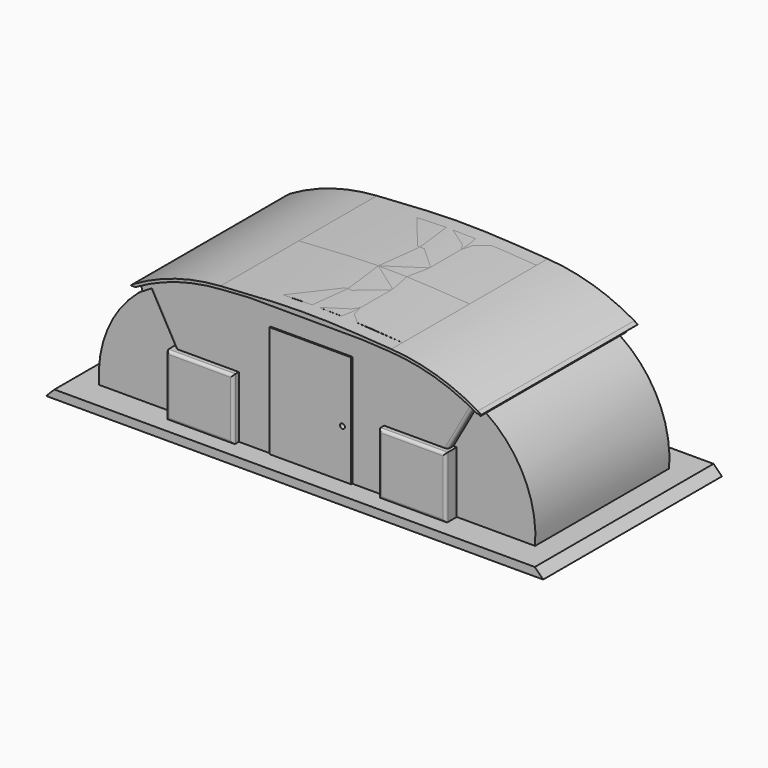
from build123d import *

# Parameters (mm, degrees)
F0_W        = 73.01958814
F0_H        = 200
F0_R        = 4.4064886868
F1_DEPTH    = 150
F2_DEPTH    = 175
F3_DEPTH    = 175
F4_DEPTH    = 162.5
F5_DEPTH    = 165
F6_R        = 5
F6_2_R      = 5
F6_3_R      = 5
F7_W        = 900
F7_H        = 400
F7_W_2      = 780.6288967379
F7_H_2      = 300
F8_DEPTH    = 15
F9_T1_DEPTH = 502.8673195186
F10_DEPTH   = 15


# Not quite as in the source:
# - a fillet or chamfer that OpenCascade refuses, or shapes differently, is made with other operations: its cross-section is extruded or revolved along the edge and cut away or added
# - ends of sketch curves that miss each other by under 0.0002 mm in the source are joined


with BuildPart() as f1:
    # F0 (on Front) → F1 (new body, symmetric)
    with BuildSketch(Plane.XZ):
        with BuildLine():
            Line((73.2485631082, 199.8381957412), (73.2485631082, -0.1618042588))
            Line((73.2485631082, -0.1618042588), (130.2289748106, -0.1618042588))
            Line((130.2289748106, -0.1618042588), (130.2289749682, 109.8381957412))
            Line((130.2289749682, 109.8381957412), (244.361110868, 109.8381957412))
            Line((244.361110868, 109.8381957412), (288.9051257209, 189.2969646801))
            ThreePointArc((288.9051257209, 189.2969646801), (295.915659625, 185.1774143178), (302.7529489944, 180.7763059474))
            Line((302.7529489944, 180.7763059474), (305.6783307484, 191.6270836714))
            ThreePointArc((305.6783307484, 191.6270836714), (230.6863223559, 224.0165542057), (150.2289749682, 238.1408019938))
            Line((150.2289749682, 238.1408019938), (102.1122379409, 240.8775282261))
            Line((102.1122379409, 240.8775282261), (-101.8451842253, 241.4292395115))
            Line((-101.8451842253, 241.4292395115), (-151.505661922, 238.0378207475))
            ThreePointArc((-151.505661922, 238.0378207475), (-231.0604446139, 223.7664550341), (-305.220380812, 191.6270836714))
            Line((-305.220380812, 191.6270836714), (-302.294999058, 180.7763059474))
            ThreePointArc((-302.294999058, 180.7763059474), (-295.4577096886, 185.1774143178), (-288.4471757845, 189.2969646801))
            Line((-288.4471757845, 189.2969646801), (-243.9031609316, 109.8381957412))
            Line((-243.9031609316, 109.8381957412), (-129.7710250318, 109.8381957412))
            Line((-129.7710250318, 109.8381957412), (-129.7710250318, -0.1618042588))
            Line((-129.7710250318, -0.1618042588), (-72.7906131718, -0.1618042588))
            Line((-72.7906131718, -0.1618042588), (-72.7906131718, 199.8381957412))
            Line((-72.7906131718, 199.8381957412), (0.2289749682, 199.8381957412))
            Line((0.2289749682, 199.8381957412), (73.2485631082, 199.8381957412))
        make_face()
        Polygon((-249.7710250318, -0.1618042588), (-129.7710250318, -0.1618042588), (-129.7710250318, 109.8381957412), (-243.9031609316, 109.8381957412), (-249.7710250318, 109.8381957412), (-249.7710250318, 46.5387346062), align=None)
        with BuildLine():
            Line((-366.9111720315, 109.3456217277), (-249.7710250318, 46.5387346062))
            Line((-249.7710250318, 46.5387346062), (-249.7710250318, 109.8381957412))
            Line((-249.7710250318, 109.8381957412), (-243.9031609316, 109.8381957412))
            Line((-243.9031609316, 109.8381957412), (-288.4471757845, 189.2969646801))
            ThreePointArc((-288.4471757845, 189.2969646801), (-295.4577096886, 185.1774143178), (-302.294999058, 180.7763059474))
            ThreePointArc((-302.294999058, 180.7763059474), (-338.967392604, 149.0089145388), (-366.9111720315, 109.3456217277))
        make_face()
        with BuildLine():
            Line((-390.0854734008, -0.1618042588), (-249.7710250318, -0.1618042588))
            Line((-249.7710250318, -0.1618042588), (-249.7710250318, 46.5387346062))
            Line((-249.7710250318, 46.5387346062), (-366.9111720315, 109.3456217277))
            ThreePointArc((-366.9111720315, 109.3456217277), (-386.3153062929, 56.2461630608), (-390.0854734008, -0.1618042588))
        make_face()
        with Locations((36.7387690382, 99.8381957412)):
            Rectangle(F0_W, F0_H)
        with Locations((57.5472824275, 86.3982066512)):
            Circle(F0_R, mode=Mode.SUBTRACT)
        with Locations((-36.2808191018, 99.8381957412)):
            Rectangle(F0_W, F0_H)
        with BuildLine():
            Line((288.9051257209, 189.2969646801), (244.361110868, 109.8381957412))
            Line((244.361110868, 109.8381957412), (250.2289749682, 109.8381957412))
            Line((250.2289749682, 109.8381957412), (250.2289749682, 46.5387346062))
            Line((250.2289749682, 46.5387346062), (367.3691219679, 109.3456217277))
            ThreePointArc((367.3691219679, 109.3456217277), (339.4253425404, 149.0089145388), (302.7529489944, 180.7763059474))
            ThreePointArc((302.7529489944, 180.7763059474), (295.915659625, 185.1774143178), (288.9051257209, 189.2969646801))
        make_face()
        with BuildLine():
            Line((250.2289749682, 46.5387346062), (250.2289749682, -0.1618042588))
            Line((250.2289749682, -0.1618042588), (390.5434233372, -0.1618042588))
            ThreePointArc((390.5434233372, -0.1618042588), (386.7732562293, 56.2461630608), (367.3691219679, 109.3456217277))
            Line((367.3691219679, 109.3456217277), (250.2289749682, 46.5387346062))
        make_face()
        with BuildLine():
            Line((130.2289749682, 109.8381957412), (130.2289749682, -0.1618042588))
            Line((130.2289749682, -0.1618042588), (190.2289749682, -0.1618042588))
            Line((190.2289749682, -0.1618042588), (191.104793533, -0.1618042588))
            Line((191.104793533, -0.1618042588), (191.104793533, 2.3381956821))
            ThreePointArc((191.104793533, 2.3381956821), (179.0104848205, 17.996944923), (197.2172556875, 25.7417641993))
            ThreePointArc((197.2172556875, 25.7417641993), (200.0262220751, 23.5936575642), (202.1212084331, 20.7448531759))
            Line((202.1212084331, 20.7448531759), (250.2289749682, 46.5387346062))
            Line((250.2289749682, 46.5387346062), (250.2289749682, 109.8381957412))
            Line((250.2289749682, 109.8381957412), (244.361110868, 109.8381957412))
            Line((244.361110868, 109.8381957412), (130.2289749682, 109.8381957412))
        make_face()
        with BuildLine():
            ThreePointArc((197.2172556875, 25.7417641993), (179.0104848205, 17.996944923), (191.104793533, 2.3381956821))
            Line((191.104793533, 2.3381956821), (191.104793533, 14.8381956821))
            Line((191.104793533, 14.8381956821), (197.2172556875, 25.7417641993))
        make_face()
        with BuildLine():
            ThreePointArc((202.1212084331, 20.7448531759), (200.0262220751, 23.5936575642), (197.2172556875, 25.7417641993))
            Line((197.2172556875, 25.7417641993), (191.104793533, 14.8381956821))
            Line((191.104793533, 14.8381956821), (202.1212084331, 20.7448531759))
        make_face()
        with BuildLine():
            Line((191.104793533, 14.8381956821), (191.104793533, 2.3381956821))
            ThreePointArc((191.104793533, 2.3381956821), (199.9436282978, 5.9993609172), (203.604793533, 14.8381956821))
            ThreePointArc((203.604793533, 14.8381956821), (203.2282251068, 17.8832583866), (202.1212084331, 20.7448531759))
            Line((202.1212084331, 20.7448531759), (191.104793533, 14.8381956821))
        make_face()
        with BuildLine():
            Line((191.104793533, 2.3381956821), (191.104793533, -0.1618043179))
            Line((191.104793533, -0.1618042588), (250.2289749682, -0.1618042588))
            Line((250.2289749682, -0.1618042588), (250.2289749682, 46.5387346062))
            Line((250.2289749682, 46.5387346062), (202.1212084331, 20.7448531759))
            ThreePointArc((202.1212084331, 20.7448531759), (203.2282251068, 17.8832583866), (203.604793533, 14.8381956821))
            ThreePointArc((203.604793533, 14.8381956821), (199.9436282978, 5.9993609172), (191.104793533, 2.3381956821))
        make_face()
        with BuildLine():
            ThreePointArc((150.2289749682, 238.1408019938), (230.6863223559, 224.0165542057), (305.6783307484, 191.6270836714))
            Line((305.6783307484, 191.6270836714), (314.0523768961, 191.6270836714))
            Line((314.0523768961, 191.6270836714), (308.1829609782, 195.9545341232))
            ThreePointArc((308.1829609782, 195.9545341232), (233.4070394956, 228.418836004), (153.1970844362, 242.9698648181))
            add(Edge.make_bspline(
                [(-152.7391344998, 242.9698648181), (-101.8451842253, 246.5544800547), (0.018788196, 253.7290685006), (102.1122379409, 246.5580511475), (153.1970844362, 242.9698648181)],
                knots=[0, 0, 0, 0, 0.4996266007, 1, 1, 1, 1], degree=3))
            ThreePointArc((-152.7391344998, 242.9698648181), (-232.9490895592, 228.418836004), (-307.7250110418, 195.9545341232))
            Line((-307.7250110418, 195.9545341232), (-313.5944269598, 191.6270836714))
            Line((-313.5944269598, 191.6270836714), (-305.220380812, 191.6270836714))
            ThreePointArc((-305.220380812, 191.6270836714), (-231.0604446139, 223.7664550341), (-151.505661922, 238.0378207475))
            Line((-151.505661922, 238.0378207475), (-101.8451842253, 241.4292395115))
            Line((-101.8451842253, 241.4292395115), (102.1122379409, 240.8775282261))
            Line((102.1122379409, 240.8775282261), (150.2289749682, 238.1408019938))
        make_face()
    extrude(amount=F1_DEPTH, both=True)


with BuildPart() as f2:
    # F0 (on Front) → F2 (new body, symmetric)
    with BuildSketch(Plane.XZ):
        with BuildLine():
            ThreePointArc((150.2289749682, 238.1408019938), (230.6863223559, 224.0165542057), (305.6783307484, 191.6270836714))
            Line((305.6783307484, 191.6270836714), (314.0523768961, 191.6270836714))
            Line((314.0523768961, 191.6270836714), (308.1829609782, 195.9545341232))
            ThreePointArc((308.1829609782, 195.9545341232), (233.4070394956, 228.418836004), (153.1970844362, 242.9698648181))
            add(Edge.make_bspline(
                [(-152.7391344998, 242.9698648181), (-101.8451842253, 246.5544800547), (0.018788196, 253.7290685006), (102.1122379409, 246.5580511475), (153.1970844362, 242.9698648181)],
                knots=[0, 0, 0, 0, 0.4996266007, 1, 1, 1, 1], degree=3))
            ThreePointArc((-152.7391344998, 242.9698648181), (-232.9490895592, 228.418836004), (-307.7250110418, 195.9545341232))
            Line((-307.7250110418, 195.9545341232), (-313.5944269598, 191.6270836714))
            Line((-313.5944269598, 191.6270836714), (-305.220380812, 191.6270836714))
            ThreePointArc((-305.220380812, 191.6270836714), (-231.0604446139, 223.7664550341), (-151.505661922, 238.0378207475))
            Line((-151.505661922, 238.0378207475), (-101.8451842253, 241.4292395115))
            Line((-101.8451842253, 241.4292395115), (102.1122379409, 240.8775282261))
            Line((102.1122379409, 240.8775282261), (150.2289749682, 238.1408019938))
        make_face()
    extrude(amount=F2_DEPTH, both=True)


with BuildPart() as f3:
    # F0 (on Front) → F3 (new body, symmetric)
    with BuildSketch(Plane.XZ):
        Polygon((-249.7710250318, -0.1618042588), (-129.7710250318, -0.1618042588), (-129.7710250318, 109.8381957412), (-243.9031609316, 109.8381957412), (-249.7710250318, 109.8381957412), (-249.7710250318, 46.5387346062), align=None)
    extrude(amount=F3_DEPTH, both=True)

    # F6#2
    f6_2_edges = [f3.edges().sort_by_distance(p)[0] for p in [
        (-189.771025, 175, -0.161804),
        (-129.771025, 175, 54.838196),
        (-189.771025, 175, 109.838196),
        (-249.771025, 175, 54.838196),
        (-189.771025, -175, -0.161804),
        (-129.771025, -175, 54.838196),
        (-189.771025, -175, 109.838196),
        (-249.771025, -175, 54.838196),
    ]]
    fillet(f6_2_edges, radius=F6_2_R)


with BuildPart() as f3b:
    # F0 (on Front) → F3, piece 2 (new body, symmetric)
    with BuildSketch(Plane.XZ):
        with BuildLine():
            Line((130.2289749682, 109.8381957412), (130.2289749682, -0.1618042588))
            Line((130.2289749682, -0.1618042588), (190.2289749682, -0.1618042588))
            Line((190.2289749682, -0.1618042588), (191.104793533, -0.1618042588))
            Line((191.104793533, -0.1618042588), (191.104793533, 2.3381956821))
            ThreePointArc((191.104793533, 2.3381956821), (179.0104848205, 17.996944923), (197.2172556875, 25.7417641993))
            ThreePointArc((197.2172556875, 25.7417641993), (200.0262220751, 23.5936575642), (202.1212084331, 20.7448531759))
            Line((202.1212084331, 20.7448531759), (250.2289749682, 46.5387346062))
            Line((250.2289749682, 46.5387346062), (250.2289749682, 109.8381957412))
            Line((250.2289749682, 109.8381957412), (244.361110868, 109.8381957412))
            Line((244.361110868, 109.8381957412), (130.2289749682, 109.8381957412))
        make_face()
        with BuildLine():
            Line((191.104793533, 2.3381956821), (191.104793533, -0.1618043179))
            Line((191.104793533, -0.1618042588), (250.2289749682, -0.1618042588))
            Line((250.2289749682, -0.1618042588), (250.2289749682, 46.5387346062))
            Line((250.2289749682, 46.5387346062), (202.1212084331, 20.7448531759))
            ThreePointArc((202.1212084331, 20.7448531759), (203.2282251068, 17.8832583866), (203.604793533, 14.8381956821))
            ThreePointArc((203.604793533, 14.8381956821), (199.9436282978, 5.9993609172), (191.104793533, 2.3381956821))
        make_face()
        with BuildLine():
            ThreePointArc((197.2172556875, 25.7417641993), (179.0104848205, 17.996944923), (191.104793533, 2.3381956821))
            Line((191.104793533, 2.3381956821), (191.104793533, 14.8381956821))
            Line((191.104793533, 14.8381956821), (197.2172556875, 25.7417641993))
        make_face()
        with BuildLine():
            Line((191.104793533, 14.8381956821), (191.104793533, 2.3381956821))
            ThreePointArc((191.104793533, 2.3381956821), (199.9436282978, 5.9993609172), (203.604793533, 14.8381956821))
            ThreePointArc((203.604793533, 14.8381956821), (203.2282251068, 17.8832583866), (202.1212084331, 20.7448531759))
            Line((202.1212084331, 20.7448531759), (191.104793533, 14.8381956821))
        make_face()
        with BuildLine():
            ThreePointArc((202.1212084331, 20.7448531759), (200.0262220751, 23.5936575642), (197.2172556875, 25.7417641993))
            Line((197.2172556875, 25.7417641993), (191.104793533, 14.8381956821))
            Line((191.104793533, 14.8381956821), (202.1212084331, 20.7448531759))
        make_face()
    extrude(amount=F3_DEPTH, both=True)

    # F6
    f6_edges = [f3b.edges().sort_by_distance(p)[0] for p in [
        (190.228975, 175, 109.838196),
        (130.228975, 175, 54.838196),
        (190.228975, 175, -0.161804),
        (250.228975, 175, 54.838196),
        (190.228975, -175, 109.838196),
        (130.228975, -175, 54.838196),
        (190.228975, -175, -0.161804),
        (250.228975, -175, 54.838196),
    ]]
    fillet(f6_edges, radius=F6_R)


with BuildPart() as f4:
    # F0 (on Front) → F4 (new body, symmetric)
    with BuildSketch(Plane.XZ):
        with Locations((-36.2808191018, 99.8381957412)):
            Rectangle(F0_W, F0_H)
        with Locations((36.7387690382, 99.8381957412)):
            Rectangle(F0_W, F0_H)
        with Locations((57.5472824275, 86.3982066512)):
            Circle(F0_R, mode=Mode.SUBTRACT)
        with BuildLine():
            Line((73.2485631082, 199.8381957412), (73.2485631082, -0.1618042588))
            Line((73.2485631082, -0.1618042588), (130.2289748106, -0.1618042588))
            Line((130.2289748106, -0.1618042588), (130.2289749682, 109.8381957412))
            Line((130.2289749682, 109.8381957412), (244.361110868, 109.8381957412))
            Line((244.361110868, 109.8381957412), (288.9051257209, 189.2969646801))
            ThreePointArc((288.9051257209, 189.2969646801), (295.915659625, 185.1774143178), (302.7529489944, 180.7763059474))
            Line((302.7529489944, 180.7763059474), (305.6783307484, 191.6270836714))
            ThreePointArc((305.6783307484, 191.6270836714), (230.6863223559, 224.0165542057), (150.2289749682, 238.1408019938))
            Line((150.2289749682, 238.1408019938), (102.1122379409, 240.8775282261))
            Line((102.1122379409, 240.8775282261), (-101.8451842253, 241.4292395115))
            Line((-101.8451842253, 241.4292395115), (-151.505661922, 238.0378207475))
            ThreePointArc((-151.505661922, 238.0378207475), (-231.0604446139, 223.7664550341), (-305.220380812, 191.6270836714))
            Line((-305.220380812, 191.6270836714), (-302.294999058, 180.7763059474))
            ThreePointArc((-302.294999058, 180.7763059474), (-295.4577096886, 185.1774143178), (-288.4471757845, 189.2969646801))
            Line((-288.4471757845, 189.2969646801), (-243.9031609316, 109.8381957412))
            Line((-243.9031609316, 109.8381957412), (-129.7710250318, 109.8381957412))
            Line((-129.7710250318, 109.8381957412), (-129.7710250318, -0.1618042588))
            Line((-129.7710250318, -0.1618042588), (-72.7906131718, -0.1618042588))
            Line((-72.7906131718, -0.1618042588), (-72.7906131718, 199.8381957412))
            Line((-72.7906131718, 199.8381957412), (0.2289749682, 199.8381957412))
            Line((0.2289749682, 199.8381957412), (73.2485631082, 199.8381957412))
        make_face()
    extrude(amount=F4_DEPTH, both=True)

    # F6#3
    f6_3_edges = [f4.edges().sort_by_distance(p)[0] for p in [
        (266.633118, 162.5, 149.56758),
        (266.633118, -162.5, 149.56758),
        (-266.175168, -162.5, 149.56758),
        (-266.175168, 162.5, 149.56758),
    ]]
    fillet(f6_3_edges, radius=F6_3_R)


with BuildPart() as f5:
    # F0 (on Front) → F5 (new body, symmetric)
    with BuildSketch(Plane.XZ):
        with Locations((-36.2808191018, 99.8381957412)):
            Rectangle(F0_W, F0_H)
        with Locations((36.7387690382, 99.8381957412)):
            Rectangle(F0_W, F0_H)
        with Locations((57.5472824275, 86.3982066512)):
            Circle(F0_R, mode=Mode.SUBTRACT)
    extrude(amount=F5_DEPTH, both=True)


with BuildPart() as f8:
    # F7 (on face) → F8 (new body)
    with BuildSketch(Plane(origin=(0, 0, -0.1618042588), x_dir=(1, 0, 0), z_dir=(0, 0, -1))):
        Rectangle(F7_W, F7_H)
        with Locations((0.2289749682, 0)):
            Rectangle(F7_W_2, F7_H_2, mode=Mode.SUBTRACT)
    extrude(amount=F8_DEPTH)

    # F9: chamfer of 20 on 2 edges, made by hand

    # F9_s2 → F9_t1 (cut)
    with BuildSketch(Plane.XZ.offset(-251.4336597593)):
        Polygon((450, -20.1618042588), (430, -0.1618042588), (450, -0.1618042588), align=None)
        Polygon((-450, -20.1618042588), (-430, -0.1618042588), (-450, -0.1618042588), align=None)
    extrude(amount=F9_T1_DEPTH, mode=Mode.SUBTRACT)


with BuildPart() as f10:
    # F10 (new): a face of the model
    f10_faces = [f1.part.faces().sort_by_distance(p)[0] for p in [
        (0.2289749682, 0, -0.1618042588),
    ]]
    extrude(f10_faces, amount=F10_DEPTH)


solid = Compound([f1.part, f2.part, f3.part, f3b.part, f4.part, f5.part, f8.part, f10.part])
